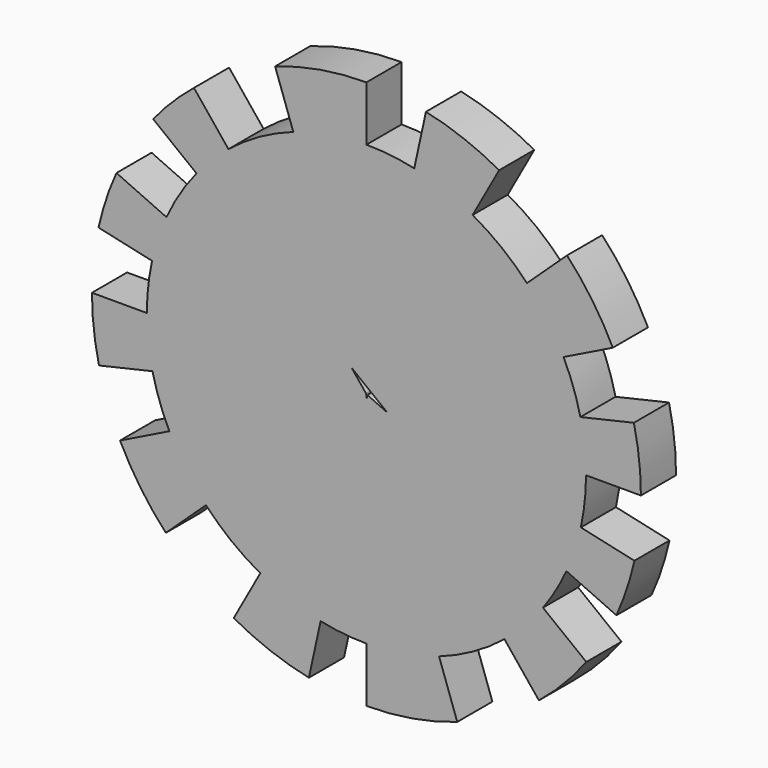
from build123d import *

# Parameters (mm, degrees)
F1_DEPTH = 5.08


with BuildPart() as f1:
    # F0 (on Front) → F1 (new body)
    with BuildSketch(Plane.XZ):
        with BuildLine():
            Line((25.4, 0), (31.75, 0))
            ThreePointArc((31.75, 0), (31.5458283638, 3.5948870413), (30.9359393487, 7.1435395019))
            Line((30.9359393487, 7.1435395019), (24.7487514789, 5.7148316015))
            ThreePointArc((24.7487514789, 5.7148316015), (25.2366626911, 2.875909633), (25.4, 0))
        make_face()
        with BuildLine():
            ThreePointArc((28.9122550087, -13.1203662416), (30.1153661217, -10.0562032277), (30.9947400528, -6.8839370321))
            Line((30.9947400528, -6.8839370321), (24.7957920422, -5.5071496257))
            ThreePointArc((24.7957920422, -5.5071496257), (24.0922928974, -8.0449625821), (23.1298040069, -10.4962929933))
            Line((23.1298040069, -10.4962929933), (28.9122550087, -13.1203662416))
        make_face()
        with BuildLine():
            ThreePointArc((24.7957920422, -5.5071496257), (25.2484961718, -2.7700976633), (25.4, 0))
            Line((25.4, 0), (1.0141198158, 0))
            Line((1.0141198158, 0), (1.4191734003, -0.3151986533))
            Line((1.4191734003, -0.3151986533), (24.7957920422, -5.5071496257))
        make_face()
        with BuildLine():
            Line((1.0141198158, 0), (25.4, 0))
            ThreePointArc((25.4, 0), (25.2366626911, 2.875909633), (24.7487514789, 5.7148316015))
            Line((24.7487514789, 5.7148316015), (0.7820524179, 0.1805868016))
            Line((0.7820524179, 0.1805868016), (1.0141198158, 0))
        make_face()
        with BuildLine():
            Line((22.7997991551, 11.1950506245), (28.4997489439, 13.9938132806))
            ThreePointArc((28.4997489439, 13.9938132806), (26.1346358015, 18.0289575828), (23.2023701208, 21.6728521606))
            Line((23.2023701208, 21.6728521606), (18.5618960967, 17.3382817285))
            ThreePointArc((18.5618960967, 17.3382817285), (20.9077086412, 14.4231660663), (22.7997991551, 11.1950506245))
        make_face()
        with BuildLine():
            Line((0.7820524179, 0.1805868016), (24.7487514789, 5.7148316015))
            ThreePointArc((24.7487514789, 5.7148316015), (23.9316603474, 8.5109125841), (22.7997991551, 11.1950506245))
            Line((22.7997991551, 11.1950506245), (0.6217813672, 0.3053041755))
            Line((0.6217813672, 0.3053041755), (0.7820524179, 0.1805868016))
        make_face()
        with BuildLine():
            ThreePointArc((23.1298040069, -10.4962929933), (24.0922928974, -8.0449625821), (24.7957920422, -5.5071496257))
            Line((24.7957920422, -5.5071496257), (1.4191734003, -0.3151986533))
            Line((1.4191734003, -0.3151986533), (2.4329098989, -1.104053243))
            Line((2.4329098989, -1.104053243), (23.1298040069, -10.4962929933))
        make_face()
        with BuildLine():
            Line((0.6217813672, 0.3053041755), (22.7997991551, 11.1950506245))
            ThreePointArc((22.7997991551, 11.1950506245), (20.9077086412, 14.4231660663), (18.5618960967, 17.3382817285))
            Line((18.5618960967, 17.3382817285), (0.4608879437, 0.4305058584))
            Line((0.4608879437, 0.4305058584), (0.6217813672, 0.3053041755))
        make_face()
        with BuildLine():
            ThreePointArc((19.9499819818, -24.6994072586), (22.8704554558, -22.02282378), (25.4348874095, -19.0033944986))
            Line((25.4348874095, -19.0033944986), (20.4222365417, -15.1027234178))
            ThreePointArc((20.4222365417, -15.1027234178), (18.3395194553, -17.5733328128), (15.9599855854, -19.7595258069))
            Line((15.9599855854, -19.7595258069), (19.9499819818, -24.6994072586))
        make_face()
        with BuildLine():
            ThreePointArc((20.4222365417, -15.1027234178), (21.8974852278, -12.8709028704), (23.1298040069, -10.4962929933))
            Line((23.1298040069, -10.4962929933), (2.4329098989, -1.104053243))
            Line((2.4329098989, -1.104053243), (20.4222365417, -15.1027234178))
        make_face()
        with BuildLine():
            Line((12.2796028487, 22.2344632019), (15.3495035609, 27.7930790024))
            ThreePointArc((15.3495035609, 27.7930790024), (11.2320077334, 29.6968769785), (6.8852258142, 30.9944537859))
            Line((6.8852258142, 30.9944537859), (5.5312442607, 24.7904283329))
            ThreePointArc((5.5312442607, 24.7904283329), (8.9966553856, 23.7533195969), (12.2796028487, 22.2344632019))
        make_face()
        with BuildLine():
            Line((0.4608879437, 0.4305058584), (18.5618960967, 17.3382817285))
            ThreePointArc((18.5618960967, 17.3382817285), (15.6138612314, 20.0341542733), (12.2796028487, 22.2344632019))
            Line((12.2796028487, 22.2344632019), (0.3048278221, 0.5519464332))
            Line((0.3048278221, 0.5519464332), (0.4608879437, 0.4305058584))
        make_face()
        with BuildLine():
            ThreePointArc((15.9599855854, -19.7595258069), (18.3395194553, -17.5733328128), (20.4222365417, -15.1027234178))
            Line((20.4222365417, -15.1027234178), (2.4329098989, -1.104053243))
            Line((2.4329098989, -1.104053243), (0.1100244544, -0.04992904))
            Line((0.1100244544, -0.04992904), (0.0951985642, -0.1178621669))
            Line((0.0951985642, -0.1178621669), (15.9599855854, -19.7595258069))
        make_face()
        with BuildLine():
            Line((0.3048278221, 0.5519464332), (12.2796028487, 22.2344632019))
            ThreePointArc((12.2796028487, 22.2344632019), (8.9966553856, 23.7533195969), (5.5312442607, 24.7904283329))
            Line((5.5312442607, 24.7904283329), (0.2505903033, 0.5941521896))
            Line((0.2505903033, 0.5941521896), (0.3048278221, 0.5519464332))
        make_face()
        with BuildLine():
            Line((0, -30.624730456), (10.5058264675, -29.9614771037))
            Line((10.5058264675, -29.9614771037), (8.3988855156, -23.9712061043))
            ThreePointArc((8.3988855156, -23.9712061043), (4.2597749325, -25.0402539429), (0, -25.4))
            Line((0, -25.4), (0, -30.624730456))
        make_face()
        with BuildLine():
            ThreePointArc((0, -31.75), (5.3284895589, -31.2996757015), (10.5058264675, -29.9614771037))
            Line((10.5058264675, -29.9614771037), (0, -30.624730456))
            Line((0, -30.624730456), (0, -31.75))
        make_face()
        with BuildLine():
            ThreePointArc((8.3988855156, -23.9712061043), (12.3601461586, -22.1897901508), (15.9599855854, -19.7595258069))
            Line((15.9599855854, -19.7595258069), (0.0951985642, -0.1178621669))
            Line((0.0951985642, -0.1178621669), (0.0621994091, -0.2690662935))
            Line((0.0621994091, -0.2690662935), (8.3988855156, -23.9712061043))
        make_face()
        with BuildLine():
            Line((-0.0300018042, -0.0069278347), (-0.0324385118, 0))
            Line((-0.0324385118, 0), (-25.4, 0))
            ThreePointArc((-25.4, 0), (-25.2366626911, -2.875909633), (-24.7487514789, -5.7148316015))
            Line((-24.7487514789, -5.7148316015), (-0.0300018042, -0.0069278347))
        make_face()
        with BuildLine():
            Line((-25.4, 0), (-0.0324385118, 0))
            Line((-0.0324385118, 0), (-0.0351872962, 0.0078151045))
            Line((-0.0351872962, 0.0078151045), (-24.7957920422, 5.5071496257))
            ThreePointArc((-24.7957920422, 5.5071496257), (-25.2484961718, 2.7700976633), (-25.4, 0))
        make_face()
        with BuildLine():
            Line((-0.03859952, 0.0175164421), (-0.0574602451, 0.0711396129))
            Line((-0.0574602451, 0.0711396129), (-1.7159178196, 2.1244206179))
            Line((-1.7159178196, 2.1244206179), (-19.6572715888, 16.085759966))
            ThreePointArc((-19.6572715888, 16.085759966), (-21.5753098418, 13.4039548354), (-23.1298040069, 10.4962929933))
            Line((-23.1298040069, 10.4962929933), (-0.03859952, 0.0175164421))
        make_face()
        with BuildLine():
            Line((0, -0.0922263513), (-0.0198174482, -0.0358831086))
            Line((-0.0198174482, -0.0358831086), (-12.2796028487, -22.2344632019))
            ThreePointArc((-12.2796028487, -22.2344632019), (-8.8860767808, -23.794907847), (-5.3003972682, -24.8408089401))
            Line((-5.3003972682, -24.8408089401), (0, -0.5540677516))
            Line((0, -0.5540677516), (0, -0.0922263513))
        make_face()
        with BuildLine():
            Line((-12.2796028487, -22.2344632019), (-0.0198174482, -0.0358831086))
            Line((-0.0198174482, -0.0358831086), (-0.0244166428, -0.0228070791))
            Line((-0.0244166428, -0.0228070791), (-18.5618960967, -17.3382817285))
            ThreePointArc((-18.5618960967, -17.3382817285), (-15.6138612314, -20.0341542733), (-12.2796028487, -22.2344632019))
        make_face()
        with BuildLine():
            Line((-0.0351872962, 0.0078151045), (-0.03859952, 0.0175164421))
            Line((-0.03859952, 0.0175164421), (-23.1298040069, 10.4962929933))
            ThreePointArc((-23.1298040069, 10.4962929933), (-24.0922928974, 8.0449625821), (-24.7957920422, 5.5071496257))
            Line((-24.7957920422, 5.5071496257), (-0.0351872962, 0.0078151045))
        make_face()
        with BuildLine():
            Line((-0.0244166428, -0.0228070791), (-0.0276613091, -0.0135821265))
            Line((-0.0276613091, -0.0135821265), (-22.7997991551, -11.1950506245))
            ThreePointArc((-22.7997991551, -11.1950506245), (-20.9077086412, -14.4231660663), (-18.5618960967, -17.3382817285))
            Line((-18.5618960967, -17.3382817285), (-0.0244166428, -0.0228070791))
        make_face()
        with BuildLine():
            Line((-22.7997991551, -11.1950506245), (-0.0276613091, -0.0135821265))
            Line((-0.0276613091, -0.0135821265), (-0.0300018042, -0.0069278347))
            Line((-0.0300018042, -0.0069278347), (-24.7487514789, -5.7148316015))
            ThreePointArc((-24.7487514789, -5.7148316015), (-23.9316603474, -8.5109125841), (-22.7997991551, -11.1950506245))
        make_face()
        with BuildLine():
            Line((-0.4268288624, 1.1212962933), (0, 0.7891528738))
            Line((0, 0.7891528738), (0, 25.4))
            ThreePointArc((0, 25.4), (-4.2899392789, 25.0351037742), (-8.4566200813, 23.95089929))
            Line((-8.4566200813, 23.95089929), (-0.4268288624, 1.1212962933))
        make_face()
        with BuildLine():
            Line((0, 25.4), (0, 0.7891528738))
            Line((0, 0.7891528738), (0.2505903033, 0.5941521896))
            Line((0.2505903033, 0.5941521896), (5.5312442607, 24.7904283329))
            ThreePointArc((5.5312442607, 24.7904283329), (2.7823659307, 25.2471471622), (0, 25.4))
        make_face()
        with BuildLine():
            Line((0, 25.4), (0, 31.75))
            ThreePointArc((0, 31.75), (-5.3586539033, 31.2945255331), (-10.5635610332, 29.9411702894))
            Line((-10.5635610332, 29.9411702894), (-8.4566200813, 23.95089929))
            ThreePointArc((-8.4566200813, 23.95089929), (-4.2899392789, 25.0351037742), (0, 25.4))
        make_face()
        with BuildLine():
            ThreePointArc((0, -25.4), (4.2597749325, -25.0402539429), (8.3988855156, -23.9712061043))
            Line((8.3988855156, -23.9712061043), (0.0621994091, -0.2690662935))
            Line((0.0621994091, -0.2690662935), (0, -0.5540677516))
            Line((0, -0.5540677516), (0, -25.4))
        make_face()
        with BuildLine():
            ThreePointArc((-24.7487514789, -5.7148316015), (-25.2366626911, -2.875909633), (-25.4, 0))
            Line((-25.4, 0), (-31.75, 0))
            ThreePointArc((-31.75, 0), (-31.5458283638, -3.5948870413), (-30.9359393487, -7.1435395019))
            Line((-30.9359393487, -7.1435395019), (-24.7487514789, -5.7148316015))
        make_face()
        with BuildLine():
            Line((-19.6572715888, 16.085759966), (-1.7159178196, 2.1244206179))
            Line((-1.7159178196, 2.1244206179), (-15.9599855854, 19.7595258069))
            ThreePointArc((-15.9599855854, 19.7595258069), (-17.9031112106, 18.017730406), (-19.6572715888, 16.085759966))
        make_face()
        with BuildLine():
            Line((-15.9599855854, 19.7595258069), (-1.7159178196, 2.1244206179))
            Line((-1.7159178196, 2.1244206179), (-0.4268288624, 1.1212962933))
            Line((-0.4268288624, 1.1212962933), (-8.4566200813, 23.95089929))
            ThreePointArc((-8.4566200813, 23.95089929), (-12.3868705083, 22.1748830664), (-15.9599855854, 19.7595258069))
        make_face()
        with BuildLine():
            ThreePointArc((-5.3003972682, -24.8408089401), (-8.8860767808, -23.794907847), (-12.2796028487, -22.2344632019))
            Line((-12.2796028487, -22.2344632019), (-15.3495035609, -27.7930790024))
            ThreePointArc((-15.3495035609, -27.7930790024), (-11.1214292363, -29.7384651881), (-6.6543788217, -31.0448343931))
            Line((-6.6543788217, -31.0448343931), (-5.3003972682, -24.8408089401))
        make_face()
        with BuildLine():
            ThreePointArc((-24.7957920422, 5.5071496257), (-24.0922928974, 8.0449625821), (-23.1298040069, 10.4962929933))
            Line((-23.1298040069, 10.4962929933), (-28.9122550087, 13.1203662416))
            ThreePointArc((-28.9122550087, 13.1203662416), (-30.1153661217, 10.0562032277), (-30.9947400528, 6.8839370321))
            Line((-30.9947400528, 6.8839370321), (-24.7957920422, 5.5071496257))
        make_face()
        with BuildLine():
            ThreePointArc((-18.5618960967, -17.3382817285), (-20.9077086412, -14.4231660663), (-22.7997991551, -11.1950506245))
            Line((-22.7997991551, -11.1950506245), (-28.4997489439, -13.9938132806))
            ThreePointArc((-28.4997489439, -13.9938132806), (-26.1346358015, -18.0289575828), (-23.2023701208, -21.6728521606))
            Line((-23.2023701208, -21.6728521606), (-18.5618960967, -17.3382817285))
        make_face()
        with BuildLine():
            Line((0, -25.4), (0, -0.5540677516))
            Line((0, -0.5540677516), (-5.3003972682, -24.8408089401))
            ThreePointArc((-5.3003972682, -24.8408089401), (-2.6649064638, -25.25981539), (0, -25.4))
        make_face()
        with BuildLine():
            ThreePointArc((-19.6572715888, 16.085759966), (-17.9031112106, 18.017730406), (-15.9599855854, 19.7595258069))
            Line((-15.9599855854, 19.7595258069), (-19.9499819818, 24.6994072586))
            ThreePointArc((-19.9499819818, 24.6994072586), (-22.4340590223, 22.4672093457), (-24.6699224566, 19.9864310467))
            Line((-24.6699224566, 19.9864310467), (-19.6572715888, 16.085759966))
        make_face()
    extrude(amount=F1_DEPTH)


solid = f1.part
